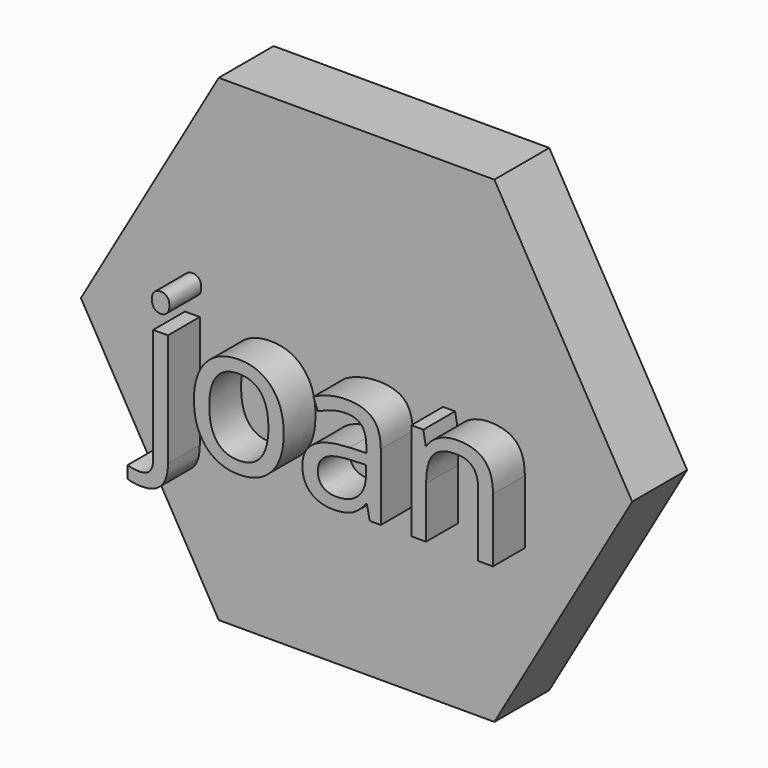
from build123d import *

# Parameters (mm, degrees)
F1_DEPTH     = 6.9
F2_TEXT_SIZE = 18.3622275169
F3_DEPTH     = 10.9


# Not quite as in the source:
# - Text() gives the source's letters only with a copy of the font that has no kerning and outlines rounded to 1/6400 em; it was checked with that copy


with BuildPart() as f1:
    # F0 (on Front) → F1 (new body)
    with BuildSketch(Plane.XZ):
        Polygon((13.855616163, 23.9986311644), (-13.855616163, 23.9986311644), (-27.7112323259, 0), (-13.855616163, -23.9986311644), (13.855616163, -23.9986311644), (27.7112323259, 0), align=None)
    extrude(amount=F1_DEPTH)

    # F2 (on Front) → F3 (join)
    with BuildSketch(Plane.XZ):
        with Locations((-18.8252758235, -7.6163327321)):
            Text('joan', F2_TEXT_SIZE, font='Open Sans', text_align=(TextAlign.LEFT, TextAlign.BOTTOM))
    extrude(amount=F3_DEPTH)


solid = f1.part
